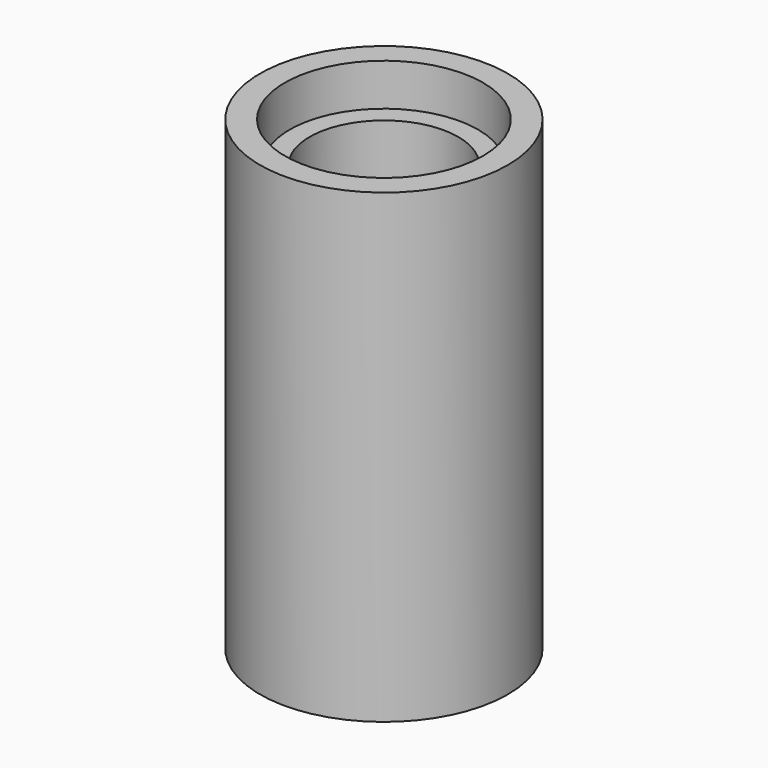
from build123d import *

# Parameters (mm, degrees)
F0_R      = 12.5
F0_R_2    = 10
F1_DEPTH  = 47
F4_T      = -2
F7_T      = -2
F9_R      = 9.5
F9_R_2    = 7.5
F10_DEPTH = 26
F11_DEPTH = 43


# Not quite as in the source:
# - a shell that OpenCascade refuses in one call is made with other operations: the cavity is built on its own and cut out


with BuildPart() as f1:
    # F0 (on Top) → F1 (new body)
    with BuildSketch(Plane.XY):
        Circle(F0_R)
        Circle(F0_R_2, mode=Mode.SUBTRACT)
    extrude(amount=F1_DEPTH)


with BuildPart() as f3:
    # F2 (on Right) → F3 (revolve)
    with BuildSketch(Plane.YZ):
        with BuildLine():
            Line((-7.5, 6), (-7.5, 0))
            Line((-7.5, 0), (0, 0))
            Line((0, 0), (0, 26))
            Line((0, 26), (-9.5, 26))
            Line((-9.5, 26), (-9.5, 11))
            add(Edge.make_bspline(
                [(-9.5, 11), (-9.4961709784, 9.3502644282), (-8.3647090448, 8.5490267521), (-7.7744109319, 7.5516820676), (-7.5, 6)],
                knots=[0, 0, 0, 0, 0.5, 1, 1, 1, 1], degree=3))
        make_face()
    revolve(axis=Axis((0, 0, 13), (0, 0, 1)))

    # F4
    f4_openings = [f3.faces().sort_by_distance(p)[0] for p in [
        (0, 0, 26),
        (0, 0, 0),
    ]]
    offset(amount=F4_T, openings=f4_openings)

    # F5 (on Right) → F6 (revolve)
    with BuildSketch(Plane.YZ):
        with BuildLine():
            Line((262.8517738675, 184.9563693243), (262.8517738675, 178.9563693243))
            Line((262.8517738675, 178.9563693243), (270.3517738675, 178.9563693243))
            Line((270.3517738675, 178.9563693243), (270.3517738675, 204.9563693243))
            Line((270.3517738675, 204.9563693243), (260.8517738675, 204.9563693243))
            Line((260.8517738675, 204.9563693243), (260.8517738675, 192.9563693243))
            add(Edge.make_bspline(
                [(260.8517738675, 192.9563693243), (261.0294527264, 189.8867335533), (261.6645518108, 189.6724810667), (263.0485391221, 186.5937816102), (262.8517738675, 184.9563693243)],
                knots=[0, 0, 0, 0, 0.5, 1, 1, 1, 1], degree=3))
        make_face()
        with BuildLine():
            Line((-7.5, 8), (-7.5, 0))
            Line((-7.5, 0), (0, 0))
            Line((0, 0), (0, 43))
            Line((0, 43), (-9.5, 43))
            Line((-9.5, 43), (-9.5, 13))
            add(Edge.make_bspline(
                [(-9.5, 13), (-9.4583500177, 11.7673277855), (-8.4318036754, 10.2421248369), (-7.6780426316, 9.7484225407), (-7.5, 8)],
                knots=[0, 0, 0, 0, 0.5, 1, 1, 1, 1], degree=3))
        make_face()
    revolve(axis=Axis((0, 0, 21.5), (0, 0, 1)))

    # F7: a shell. OpenCascade refuses it in one call, so the cavity is built on its own and cut out:
    # the body offset inwards by the wall thickness, plus a prism from it out through each open face.
    f7_core = offset(f3.part, amount=F7_T, mode=Mode.PRIVATE)
    f7_exits = [f7_core.faces().sort_by_distance(p)[0] for p in [
        (0, 0, 41),
        (0, 0, 2),
    ]]
    add(f7_core, mode=Mode.SUBTRACT)
    extrude(f7_exits, amount=-F7_T, mode=Mode.SUBTRACT)


with BuildPart() as f10:
    # F9 (on Top) → F10 (new body)
    with BuildSketch(Plane.XY):
        Circle(F9_R)
        Circle(F9_R_2, mode=Mode.SUBTRACT)
    extrude(amount=F10_DEPTH)


with BuildPart() as f11:
    # F9 (on Top) → F11 (new body)
    with BuildSketch(Plane.XY):
        Circle(F9_R)
        Circle(F9_R_2, mode=Mode.SUBTRACT)
    extrude(amount=F11_DEPTH)


solid = Compound([f1.part, f10.part, f11.part])
